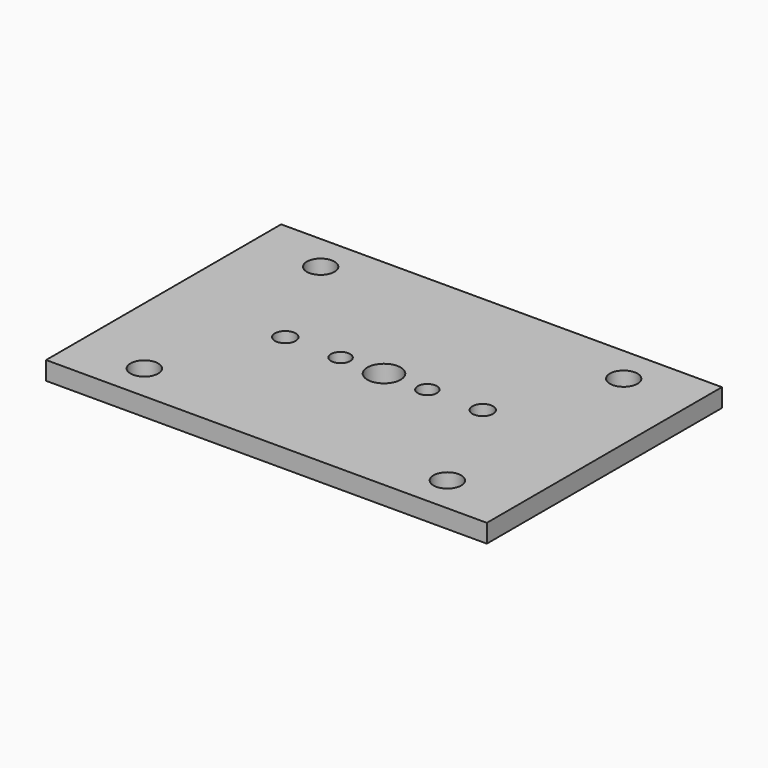
from build123d import *

# Parameters (mm, degrees)
F0_W     = 152.4
F0_H     = 101.6
F1_DEPTH = 6.35
F2_R     = 4.78155
F3_DEPTH = 6.35
F5_DEPTH = 6.351
F6_R     = 3.3
F7_DEPTH = 6.351
F9_D     = 11.50874


with BuildPart() as f1:
    # F0 (on Top) → F1 (new body)
    with BuildSketch(Plane.XY):
        Rectangle(F0_W, F0_H)
    extrude(amount=F1_DEPTH)

    # F2 (on face) → F3 (cut, through all)
    with BuildSketch(Plane.XY.offset(6.35)):
        with Locations((-52.3875, 38.1)):
            Circle(F2_R)
        with Locations((52.3875, 38.1)):
            Circle(F2_R)
        with Locations((-52.3875, -38.1)):
            Circle(F2_R)
        with Locations((52.3875, -38.1)):
            Circle(F2_R)
    extrude(amount=-F3_DEPTH, mode=Mode.SUBTRACT)

    # F4 (on face) → F5 (cut, through all)
    with BuildSketch(Plane.XY.offset(6.35)):
        with BuildLine():
            Line((-34.2171942442, -3.5708408817), (-34.13125, -3.571875))
            ThreePointArc((-34.13125, -3.571875), (-34.0882747673, 3.5716164611), (-34.2171942442, -3.5708408817))
        make_face()
        with BuildLine():
            Line((34.13125, -3.571875), (34.2751243473, -3.56897621))
            ThreePointArc((34.2751243473, -3.56897621), (34.0592982266, 3.571150229), (34.13125, -3.571875))
        make_face()
    extrude(amount=-F5_DEPTH, mode=Mode.SUBTRACT)

    # F6 (on face) → F7 (cut, through all)
    with BuildSketch(Plane.XY.offset(6.35)):
        with Locations((-15, 0)):
            Circle(F6_R)
        with Locations((15, 0)):
            Circle(F6_R)
    extrude(amount=-F7_DEPTH, mode=Mode.SUBTRACT)

    # F9 (through all)
    with Locations(Plane(origin=(0, 0, 0), x_dir=(1, 0, 0), z_dir=(0, 0, -1))):
        with Locations((0, 0)):
            Hole(F9_D / 2)


solid = f1.part
